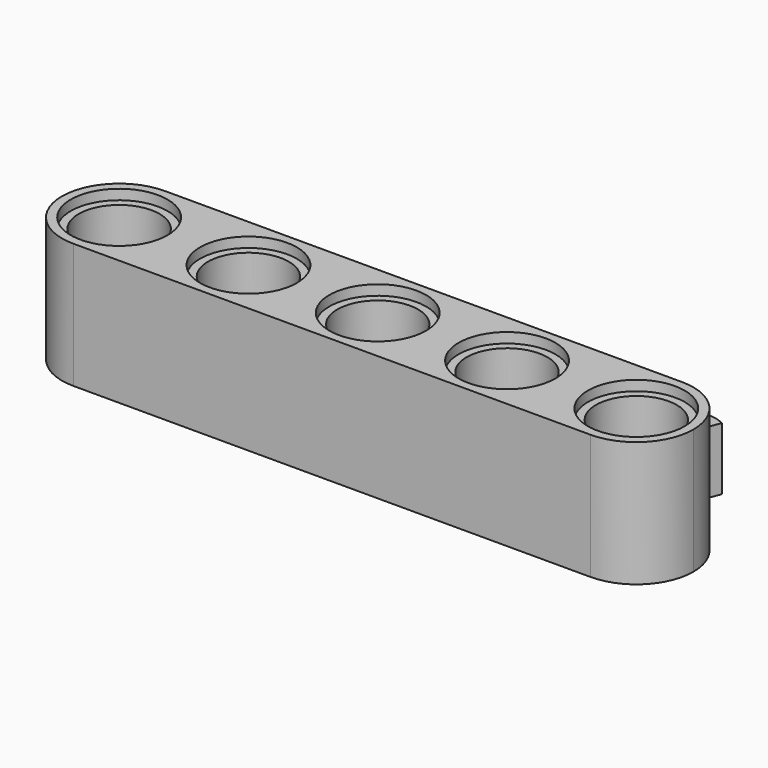
from build123d import *

# Parameters (mm, degrees)
F0_R         = 3.048
F0_R_2       = 2.54
F1_DEPTH     = 3.937
F2_R         = 3.0417071759
F3_DEPTH     = 0.635
F4_R         = 3.048
F5_DEPTH     = 0.635
F6_TEXT_SIZE = 7.5637000716
F7_DEPTH     = 3.937
F8_SIZE2     = 0.50799
F8_SIZE      = 0.50799
F9_SIZE2     = 0.50799
F9_SIZE      = 0.50799


# Not quite as in the source:
# - a fillet or chamfer is up to 0.001 mm smaller than in the source, because OpenCascade refuses the exact size
# - Text() gives the source's letters only with a copy of the font that has no kerning and outlines rounded to 1/6400 em; it was checked with that copy


with BuildPart() as f1:
    # F0 (on Top) → F1 (new body, symmetric)
    with BuildSketch(Plane.XY):
        with BuildLine():
            ThreePointArc((-40.9946195992, 14.3710068385), (-42.0464330806, 16.9103092103), (-44.5857354524, 17.9621226917))
            ThreePointArc((-44.5857354524, 17.9621226917), (-48.1768513056, 14.3710068385), (-44.5857354524, 10.7798909853))
            ThreePointArc((-44.5857354524, 10.7798909853), (-42.0464330806, 11.8317044667), (-40.9946195992, 14.3710068385))
        make_face()
        with Locations((-44.5857354524, 14.3710068385)):
            Circle(F0_R, mode=Mode.SUBTRACT)
        with BuildLine():
            ThreePointArc((-49.1226195992, 14.3710068385), (-50.1744330806, 16.9103092103), (-52.7137354524, 17.9621226917))
            ThreePointArc((-52.7137354524, 17.9621226917), (-56.3048513056, 14.3710068385), (-52.7137354524, 10.7798909853))
            ThreePointArc((-52.7137354524, 10.7798909853), (-50.1744330806, 11.8317044667), (-49.1226195992, 14.3710068385))
        make_face()
        with Locations((-52.7137354524, 14.3710068385)):
            Circle(F0_R, mode=Mode.SUBTRACT)
        with BuildLine():
            ThreePointArc((-32.8666195992, 14.3710068385), (-33.9184330806, 16.9103092103), (-36.4577354524, 17.9621226917))
            ThreePointArc((-36.4577354524, 17.9621226917), (-40.0488513056, 14.3710068385), (-36.4577354524, 10.7798909853))
            ThreePointArc((-36.4577354524, 10.7798909853), (-33.9184330806, 11.8317044667), (-32.8666195992, 14.3710068385))
        make_face()
        with Locations((-36.4577354524, 14.3710068385)):
            Circle(F0_R, mode=Mode.SUBTRACT)
        with BuildLine():
            ThreePointArc((-24.7386195992, 14.3710068385), (-25.7904330806, 16.9103092103), (-28.3297354524, 17.9621226917))
            ThreePointArc((-28.3297354524, 17.9621226917), (-31.9208513056, 14.3710068385), (-28.3297354524, 10.7798909853))
            ThreePointArc((-28.3297354524, 10.7798909853), (-25.7904330806, 11.8317044667), (-24.7386195992, 14.3710068385))
        make_face()
        with Locations((-28.3297354524, 14.3710068385)):
            Circle(F0_R, mode=Mode.SUBTRACT)
        with BuildLine():
            ThreePointArc((-60.8417354524, 10.7798909853), (-58.3024330806, 11.8317044667), (-57.2506195992, 14.3710068385))
            ThreePointArc((-57.2506195992, 14.3710068385), (-58.3024330806, 16.9103092103), (-60.8417354524, 17.9621226917))
            ThreePointArc((-60.8417354524, 17.9621226917), (-64.4328513056, 14.3710068385), (-60.8417354524, 10.7798909853))
        make_face()
        with Locations((-60.8417354524, 14.3710068385)):
            Circle(F0_R, mode=Mode.SUBTRACT)
        with Locations((-44.5857354524, 14.3710068385)):
            Circle(F0_R)
        with Locations((-44.5857354524, 14.3710068385)):
            Circle(F0_R_2, mode=Mode.SUBTRACT)
        with Locations((-36.4577354524, 14.3710068385)):
            Circle(F0_R)
        with Locations((-36.4577354524, 14.3710068385)):
            Circle(F0_R_2, mode=Mode.SUBTRACT)
        with Locations((-52.7137354524, 14.3710068385)):
            Circle(F0_R)
        with Locations((-52.7137354524, 14.3710068385)):
            Circle(F0_R_2, mode=Mode.SUBTRACT)
        with Locations((-28.3297354524, 14.3710068385)):
            Circle(F0_R)
        with Locations((-28.3297354524, 14.3710068385)):
            Circle(F0_R_2, mode=Mode.SUBTRACT)
        with Locations((-60.8417354524, 14.3710068385)):
            Circle(F0_R)
        with Locations((-60.8417354524, 14.3710068385)):
            Circle(F0_R_2, mode=Mode.SUBTRACT)
        with BuildLine():
            ThreePointArc((-60.8417354524, 17.9621226917), (-58.3024330806, 16.9103092103), (-57.2506195992, 14.3710068385))
            ThreePointArc((-57.2506195992, 14.3710068385), (-58.3024330806, 11.8317044667), (-60.8417354524, 10.7798909853))
            Line((-60.8417354524, 10.7798909853), (-52.7137354524, 10.7798909853))
            ThreePointArc((-52.7137354524, 10.7798909853), (-56.3048513056, 14.3710068385), (-52.7137354524, 17.9621226917))
            Line((-52.7137354524, 17.9621226917), (-60.8417354524, 17.9621226917))
        make_face()
        with BuildLine():
            Line((-44.5857354524, 17.9621226917), (-52.7137354524, 17.9621226917))
            ThreePointArc((-52.7137354524, 17.9621226917), (-50.1744330806, 16.9103092103), (-49.1226195992, 14.3710068385))
            ThreePointArc((-49.1226195992, 14.3710068385), (-50.1744330806, 11.8317044667), (-52.7137354524, 10.7798909853))
            Line((-52.7137354524, 10.7798909853), (-44.5857354524, 10.7798909853))
            ThreePointArc((-44.5857354524, 10.7798909853), (-48.1768513056, 14.3710068385), (-44.5857354524, 17.9621226917))
        make_face()
        with BuildLine():
            Line((-28.3297354524, 17.9621226917), (-36.4577354524, 17.9621226917))
            ThreePointArc((-36.4577354524, 17.9621226917), (-33.9184330806, 16.9103092103), (-32.8666195992, 14.3710068385))
            ThreePointArc((-32.8666195992, 14.3710068385), (-33.9184330806, 11.8317044667), (-36.4577354524, 10.7798909853))
            Line((-36.4577354524, 10.7798909853), (-28.3297354524, 10.7798909853))
            ThreePointArc((-28.3297354524, 10.7798909853), (-31.9208513056, 14.3710068385), (-28.3297354524, 17.9621226917))
        make_face()
        with BuildLine():
            Line((-36.4577354524, 17.9621226917), (-44.5857354524, 17.9621226917))
            ThreePointArc((-44.5857354524, 17.9621226917), (-42.0464330806, 16.9103092103), (-40.9946195992, 14.3710068385))
            ThreePointArc((-40.9946195992, 14.3710068385), (-42.0464330806, 11.8317044667), (-44.5857354524, 10.7798909853))
            Line((-44.5857354524, 10.7798909853), (-36.4577354524, 10.7798909853))
            ThreePointArc((-36.4577354524, 10.7798909853), (-40.0488513056, 14.3710068385), (-36.4577354524, 17.9621226917))
        make_face()
    extrude(amount=F1_DEPTH, both=True)

    # F2 (on face) → F3 (cut)
    with BuildSketch(Plane.XY.offset(3.937)):
        with Locations((-28.3297354524, 14.3710068385)):
            Circle(F2_R)
        with Locations((-36.4577354524, 14.3710068385)):
            Circle(F2_R)
        with Locations((-44.5857354524, 14.3710068385)):
            Circle(F2_R)
        with Locations((-52.7137354524, 14.3710068385)):
            Circle(F2_R)
        with Locations((-60.8417354524, 14.3710068385)):
            Circle(F2_R)
    extrude(amount=-F3_DEPTH, mode=Mode.SUBTRACT)

    # F4 (on face) → F5 (cut)
    with BuildSketch(Plane(origin=(0, 0, -3.937), x_dir=(1, 0, 0), z_dir=(0, 0, -1))):
        with Locations((-60.8417354524, -14.3710068385)):
            Circle(F4_R)
        with Locations((-52.7137354524, -14.3710068385)):
            Circle(F4_R)
        with Locations((-44.5857354524, -14.3710068385)):
            Circle(F4_R)
        with Locations((-36.4577354524, -14.3710068385)):
            Circle(F4_R)
        with Locations((-28.3297354524, -14.3710068385)):
            Circle(F4_R)
    extrude(amount=-F5_DEPTH, mode=Mode.SUBTRACT)

    # F6 (on Top) → F7 (join)
    with BuildSketch(Plane.XY):
        with Locations((-60.9262157232, 17.7584644407)):
            Text('bazmarc', F6_TEXT_SIZE, font='Open Sans', font_style=FontStyle.BOLD, text_align=(TextAlign.LEFT, TextAlign.BOTTOM))
    extrude(amount=-F7_DEPTH)

    # F8 (size 0.508 and 0.508 in the source; OpenCascade refuses exactly that, so slightly less here)
    f8_edges = [f1.edges().sort_by_distance(p)[0] for p in [
        (-38.997735, 14.371007, -3.302),
    ]]
    chamfer(f8_edges, length=F8_SIZE, length2=F8_SIZE2)

    # F9 (size 0.508 and 0.508 in the source; OpenCascade refuses exactly that, so slightly less here)
    f9_edges = [f1.edges().sort_by_distance(p)[0] for p in [
        (-47.125735, 14.371007, -3.302),
        (-55.253735, 14.371007, -3.302),
        (-63.381735, 14.371007, -3.302),
        (-30.869735, 14.371007, -3.302),
    ]]
    chamfer(f9_edges, length=F9_SIZE, length2=F9_SIZE2)


solid = f1.part
